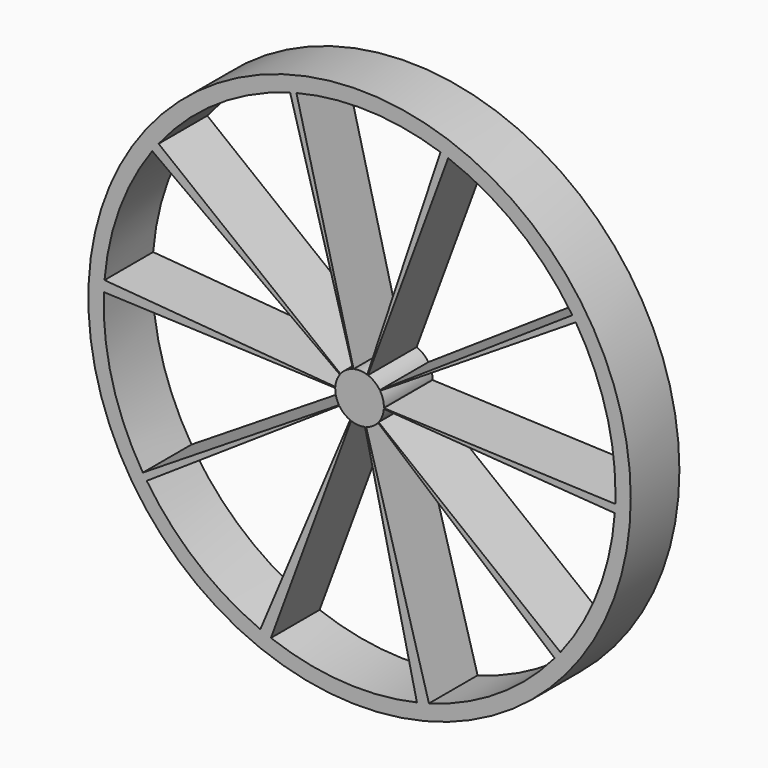
from build123d import *

# Parameters (mm, degrees)
F1_DEPTH = 25.4
F0_R     = 113.2713200319
F2_DEPTH = 25.4


with BuildPart() as f1:
    # F0 (on Front) → F1 (new body)
    with BuildSketch(Plane.XZ):
        with BuildLine():
            Line((0, 0), (8.4491764715, 5.6424300575))
            ThreePointArc((8.4491764715, 5.6424300575), (6.2920375632, 7.9772089921), (3.518990179, 9.53112313))
            Line((3.518990179, 9.53112313), (0, 0))
        make_face()
        with BuildLine():
            Line((-2.5059085691, 9.8461171151), (0, 0))
            Line((0, 0), (3.2131374582, 9.6385345191))
            ThreePointArc((3.2131374582, 9.6385345191), (0.3685319646, 10.1533139512), (-2.5059085691, 9.8461171151))
        make_face()
        with BuildLine():
            Line((-7.9772089921, 6.2920375632), (0, 0))
            Line((0, 0), (-2.7553307558, 9.7792511179))
            ThreePointArc((-2.7553307558, 9.7792511179), (-5.6424300575, 8.4491764715), (-7.9772089921, 6.2920375632))
        make_face()
        with BuildLine():
            Line((-10.1262826145, 0.8270431738), (0, 0))
            Line((0, 0), (-8.2305254154, 5.9568491156))
            ThreePointArc((-8.2305254154, 5.9568491156), (-9.5300486626, 3.5218989889), (-10.1262826145, 0.8270431738))
        make_face()
        with BuildLine():
            Line((-8.6028237663, -5.4052773514), (0, 0))
            Line((0, 0), (-10.1520645288, 0.4014795179))
            ThreePointArc((-10.1520645288, 0.4014795179), (-9.816621877, -2.619071386), (-8.6028237663, -5.4052773514))
        make_face()
        with BuildLine():
            Line((2.2787747925, -9.9011507132), (0, 0))
            Line((0, 0), (-3.518990179, -9.53112313))
            ThreePointArc((-3.518990179, -9.53112313), (-0.6471195054, -10.139370609), (2.2787747925, -9.9011507132))
        make_face()
        with BuildLine():
            Line((7.7452963463, -6.5754075545), (0, 0))
            Line((0, 0), (2.7553307558, -9.7792511179))
            ThreePointArc((2.7553307558, -9.7792511179), (5.4892573067, -8.5494826873), (7.7452963463, -6.5754075545))
        make_face()
        with BuildLine():
            Line((10.1339284401, -0.727388734), (0, 0))
            Line((0, 0), (7.9772089921, -6.2920375632))
            ThreePointArc((7.9772089921, -6.2920375632), (9.4733655012, -3.6716407885), (10.1339284401, -0.727388734))
        make_face()
        with BuildLine():
            Line((-2.7553307558, 9.7792511179), (0, 0))
            Line((0, 0), (-2.5059085691, 9.8461171151))
            ThreePointArc((-2.5059085691, 9.8461171151), (-2.6308321067, 9.8134765719), (-2.7553307558, 9.7792511179))
        make_face()
        with BuildLine():
            Line((-8.2305254154, 5.9568491156), (0, 0))
            Line((0, 0), (-7.9772089921, 6.2920375632))
            ThreePointArc((-7.9772089921, 6.2920375632), (-8.1056000074, 6.1257528942), (-8.2305254154, 5.9568491156))
        make_face()
        with BuildLine():
            Line((-10.1520645288, 0.4014795179), (0, 0))
            Line((0, 0), (-10.1262826145, 0.8270431738))
            ThreePointArc((-10.1262826145, 0.8270431738), (-10.1414060575, 0.6143965965), (-10.1520645288, 0.4014795179))
        make_face()
        with BuildLine():
            Line((-8.4491764715, -5.6424300575), (0, 0))
            Line((0, 0), (-8.6028237663, -5.4052773514))
            ThreePointArc((-8.6028237663, -5.4052773514), (-8.5268246363, -5.5243878956), (-8.4491764715, -5.6424300575))
        make_face()
        with BuildLine():
            Line((-3.9385917856, -9.3655269337), (0, 0))
            Line((0, 0), (-8.4491764715, -5.6424300575))
            ThreePointArc((-8.4491764715, -5.6424300575), (-6.4675778453, -7.8355623164), (-3.9385917856, -9.3655269337))
        make_face()
        with BuildLine():
            Line((2.7553307558, -9.7792511179), (0, 0))
            Line((0, 0), (2.2787747925, -9.9011507132))
            ThreePointArc((2.2787747925, -9.9011507132), (2.517790608, -9.8430854133), (2.7553307558, -9.7792511179))
        make_face()
        with BuildLine():
            Line((-3.518990179, -9.53112313), (0, 0))
            Line((0, 0), (-3.9385917856, -9.3655269337))
            ThreePointArc((-3.9385917856, -9.3655269337), (-3.7297101382, -9.4506540665), (-3.518990179, -9.53112313))
        make_face()
        with BuildLine():
            Line((7.9772089921, -6.2920375632), (0, 0))
            Line((0, 0), (7.7452963463, -6.5754075545))
            ThreePointArc((7.7452963463, -6.5754075545), (7.8625293746, -6.4347674265), (7.9772089921, -6.2920375632))
        make_face()
        with BuildLine():
            ThreePointArc((10.1339284401, -0.727388734), (10.1443053921, -0.5645069636), (10.1520645288, -0.4014795179))
            Line((10.1520645288, -0.4014795179), (0, 0))
            Line((0, 0), (10.1339284401, -0.727388734))
        make_face()
        with BuildLine():
            ThreePointArc((10.1520645288, -0.4014795179), (10.1580159385, -0.2007789674), (10.16, 0))
            ThreePointArc((10.16, 0), (9.7577263861, 2.8306140277), (8.5827606744, 5.4370781864))
            Line((8.5827606744, 5.4370781864), (0, 0))
            Line((0, 0), (10.1520645288, -0.4014795179))
        make_face()
        with BuildLine():
            Line((0, 0), (8.5827606744, 5.4370781864))
            ThreePointArc((8.5827606744, 5.4370781864), (8.5165875257, 5.5401567592), (8.4491764715, 5.6424300575))
            Line((8.4491764715, 5.6424300575), (0, 0))
        make_face()
        with BuildLine():
            Line((3.2131374582, 9.6385345191), (0, 0))
            Line((0, 0), (3.518990179, 9.53112313))
            ThreePointArc((3.518990179, 9.53112313), (3.3664922297, 9.5860487203), (3.2131374582, 9.6385345191))
        make_face()
    extrude(amount=F1_DEPTH)

    # F0 (on Front) → F2 (join)
    with BuildSketch(Plane.XZ):
        Circle(F0_R)
        Polygon((90.5068083934, 60.4411965841), (91.6145348169, 58.0367329004), (104.7544467964, 29.5148519638), (108.7479900799, -4.3006120088), (108.0596985006, -7.7562623179), (102.0965224025, -37.6951021138), (85.4511357641, -67.3997329867), (60.4411965841, -90.5068083934), (29.5148519638, -104.7544467964), (-4.3006120088, -108.7479900799), (-37.6951021138, -102.0965224025), (-67.3997329867, -85.4511357641), (-90.5068083934, -60.4411965841), (-91.7838875883, -57.669130774), (-104.7544467964, -29.5148519638), (-108.7479900799, 4.3006120088), (-107.850128026, 8.8084359851), (-102.0965224025, 37.6951021138), (-87.6655406442, 63.4480026369), (-85.4511357641, 67.3997329867), (-60.4411965841, 90.5068083934), (-29.5148519638, 104.7544467964), (-26.7440517016, 105.0816731443), (4.3006120088, 108.7479900799), (34.2631514946, 102.7800935109), (37.6951021138, 102.0965224025), (67.3997329867, 85.4511357641), align=None, mode=Mode.SUBTRACT)
        with BuildLine():
            ThreePointArc((-8.2305254154, 5.9568491156), (-8.1056000074, 6.1257528942), (-7.9772089921, 6.2920375632))
            Line((-7.9772089921, 6.2920375632), (-83.9123738102, 66.1860318007))
            ThreePointArc((-83.9123738102, 66.1860318007), (-85.2629207095, 64.4368810237), (-86.577012837, 62.6601797971))
            Line((-86.577012837, 62.6601797971), (-8.2305254154, 5.9568491156))
        make_face()
        with BuildLine():
            Line((-28.9833630506, 102.8680803274), (-2.7553307558, 9.7792511179))
            ThreePointArc((-2.7553307558, 9.7792511179), (-2.6308321067, 9.8134765719), (-2.5059085691, 9.8461171151))
            Line((-2.5059085691, 9.8461171151), (-26.3596875538, 103.5714446942))
            ThreePointArc((-26.3596875538, 103.5714446942), (-27.6737600067, 103.2280983602), (-28.9833630506, 102.8680803274))
        make_face()
        with BuildLine():
            ThreePointArc((3.2131374582, 9.6385345191), (3.3664922297, 9.5860487203), (3.518990179, 9.53112313))
            Line((3.518990179, 9.53112313), (37.0163072861, 100.2580185266))
            ThreePointArc((37.0163072861, 100.2580185266), (35.4121792077, 100.8357815844), (33.7990382049, 101.3878804414))
            Line((33.7990382049, 101.3878804414), (3.2131374582, 9.6385345191))
        make_face()
        with BuildLine():
            ThreePointArc((8.4491764715, 5.6424300575), (8.5165875257, 5.5401567592), (8.5827606744, 5.4370781864))
            Line((8.5827606744, 5.4370781864), (90.282180491, 57.1927020673))
            ThreePointArc((90.282180491, 57.1927020673), (89.5861042071, 58.2769870272), (88.8770063774, 59.3528012933))
            Line((88.8770063774, 59.3528012933), (8.4491764715, 5.6424300575))
        make_face()
        with BuildLine():
            Line((106.789709851, -4.2231687065), (10.1520645288, -0.4014795179))
            ThreePointArc((10.1520645288, -0.4014795179), (10.1443053921, -0.5645069636), (10.1339284401, -0.727388734))
            Line((10.1339284401, -0.727388734), (106.5989360787, -7.6514123443))
            ThreePointArc((106.5989360787, -7.6514123443), (106.7080913827, -5.9380567058), (106.789709851, -4.2231687065))
        make_face()
        with BuildLine():
            Line((83.9123738102, -66.1860318007), (7.9772089921, -6.2920375632))
            ThreePointArc((7.9772089921, -6.2920375632), (7.8625293746, -6.4347674265), (7.7452963463, -6.5754075545))
            Line((7.7452963463, -6.5754075545), (81.4728814213, -69.1668047323))
            ThreePointArc((81.4728814213, -69.1668047323), (82.7060572982, -67.687409244), (83.9123738102, -66.1860318007))
        make_face()
        with BuildLine():
            Line((28.9833630506, -102.8680803274), (2.7553307558, -9.7792511179))
            ThreePointArc((2.7553307558, -9.7792511179), (2.517790608, -9.8430854133), (2.2787747925, -9.9011507132))
            Line((2.2787747925, -9.9011507132), (23.9704641575, -104.1503438883))
            ThreePointArc((23.9704641575, -104.1503438883), (26.4846748886, -103.5395541811), (28.9833630506, -102.8680803274))
        make_face()
        with BuildLine():
            Line((-37.0163072861, -100.2580185266), (-3.518990179, -9.53112313))
            ThreePointArc((-3.518990179, -9.53112313), (-3.7297101382, -9.4506540665), (-3.9385917856, -9.3655269337))
            Line((-3.9385917856, -9.3655269337), (-41.4301024994, -98.5161098038))
            ThreePointArc((-41.4301024994, -98.5161098038), (-39.2328735062, -99.4115633134), (-37.0163072861, -100.2580185266))
        make_face()
        with BuildLine():
            Line((-88.8770063774, -59.3528012933), (-8.4491764715, -5.6424300575))
            ThreePointArc((-8.4491764715, -5.6424300575), (-8.5268246363, -5.5243878956), (-8.6028237663, -5.4052773514))
            Line((-8.6028237663, -5.4052773514), (-90.4932244371, -56.8581886358))
            ThreePointArc((-90.4932244371, -56.8581886358), (-89.6937885179, -58.1111141287), (-88.8770063774, -59.3528012933))
        make_face()
        with BuildLine():
            Line((-106.789709851, 4.2231687065), (-10.1520645288, 0.4014795179))
            ThreePointArc((-10.1520645288, 0.4014795179), (-10.1414060575, 0.6143965965), (-10.1262826145, 0.8270431738))
            Line((-10.1262826145, 0.8270431738), (-106.5185095312, 8.6996788006))
            ThreePointArc((-106.5185095312, 8.6996788006), (-106.6775932408, 6.462846457), (-106.789709851, 4.2231687065))
        make_face()
        with BuildLine():
            ThreePointArc((-86.577012837, 62.6601797971), (-85.2629207095, 64.4368810237), (-83.9123738102, 66.1860318007))
            Line((-83.9123738102, 66.1860318007), (-85.4511357641, 67.3997329867))
            Line((-85.4511357641, 67.3997329867), (-87.6655406442, 63.4480026369))
            Line((-87.6655406442, 63.4480026369), (-86.577012837, 62.6601797971))
        make_face()
        with BuildLine():
            Line((-108.7479900799, 4.3006120088), (-106.789709851, 4.2231687065))
            ThreePointArc((-106.789709851, 4.2231687065), (-106.6775932408, 6.462846457), (-106.5185095312, 8.6996788006))
            Line((-106.5185095312, 8.6996788006), (-107.850128026, 8.8084359851))
            Line((-107.850128026, 8.8084359851), (-108.7479900799, 4.3006120088))
        make_face()
        with BuildLine():
            ThreePointArc((-106.5185095312, 8.6996788006), (-100.2467161886, 37.0469050984), (-86.577012837, 62.6601797971))
            Line((-86.577012837, 62.6601797971), (-87.6655406442, 63.4480026369))
            Line((-87.6655406442, 63.4480026369), (-102.0965224025, 37.6951021138))
            Line((-102.0965224025, 37.6951021138), (-107.850128026, 8.8084359851))
            Line((-107.850128026, 8.8084359851), (-106.5185095312, 8.6996788006))
        make_face()
        with BuildLine():
            Line((-91.7838875883, -57.669130774), (-90.4932244371, -56.8581886358))
            ThreePointArc((-90.4932244371, -56.8581886358), (-103.261183869, -27.5500488194), (-106.789709851, 4.2231687065))
            Line((-106.789709851, 4.2231687065), (-108.7479900799, 4.3006120088))
            Line((-108.7479900799, 4.3006120088), (-104.7544467964, -29.5148519638))
            Line((-104.7544467964, -29.5148519638), (-91.7838875883, -57.669130774))
        make_face()
        with BuildLine():
            Line((-90.5068083934, -60.4411965841), (-88.8770063774, -59.3528012933))
            ThreePointArc((-88.8770063774, -59.3528012933), (-89.6937885179, -58.1111141287), (-90.4932244371, -56.8581886358))
            Line((-90.4932244371, -56.8581886358), (-91.7838875883, -57.669130774))
            Line((-91.7838875883, -57.669130774), (-90.5068083934, -60.4411965841))
        make_face()
        with BuildLine():
            Line((-37.6951021138, -102.0965224025), (-37.0163072861, -100.2580185266))
            ThreePointArc((-37.0163072861, -100.2580185266), (-39.2328735062, -99.4115633134), (-41.4301024994, -98.5161098038))
            ThreePointArc((-41.4301024994, -98.5161098038), (-68.0325425023, -82.4223904327), (-88.8770063774, -59.3528012933))
            Line((-88.8770063774, -59.3528012933), (-90.5068083934, -60.4411965841))
            Line((-90.5068083934, -60.4411965841), (-67.3997329867, -85.4511357641))
            Line((-67.3997329867, -85.4511357641), (-37.6951021138, -102.0965224025))
        make_face()
        with BuildLine():
            Line((29.5148519638, -104.7544467964), (28.9833630506, -102.8680803274))
            ThreePointArc((28.9833630506, -102.8680803274), (26.4846748886, -103.5395541811), (23.9704641575, -104.1503438883))
            ThreePointArc((23.9704641575, -104.1503438883), (-6.8070591972, -106.6561823293), (-37.0163072861, -100.2580185266))
            Line((-37.0163072861, -100.2580185266), (-37.6951021138, -102.0965224025))
            Line((-37.6951021138, -102.0965224025), (-4.3006120088, -108.7479900799))
            Line((-4.3006120088, -108.7479900799), (29.5148519638, -104.7544467964))
        make_face()
        with BuildLine():
            Line((85.4511357641, -67.3997329867), (83.9123738102, -66.1860318007))
            ThreePointArc((83.9123738102, -66.1860318007), (82.7060572982, -67.687409244), (81.4728814213, -69.1668047323))
            ThreePointArc((81.4728814213, -69.1668047323), (57.7415749689, -89.9321288755), (28.9833630506, -102.8680803274))
            Line((28.9833630506, -102.8680803274), (29.5148519638, -104.7544467964))
            Line((29.5148519638, -104.7544467964), (60.4411965841, -90.5068083934))
            Line((60.4411965841, -90.5068083934), (85.4511357641, -67.3997329867))
        make_face()
        with BuildLine():
            Line((108.0596985006, -7.7562623179), (106.5989360787, -7.6514123443))
            ThreePointArc((106.5989360787, -7.6514123443), (99.6504652153, -38.6220411987), (83.9123738102, -66.1860318007))
            Line((83.9123738102, -66.1860318007), (85.4511357641, -67.3997329867))
            Line((85.4511357641, -67.3997329867), (102.0965224025, -37.6951021138))
            Line((102.0965224025, -37.6951021138), (108.0596985006, -7.7562623179))
        make_face()
        with BuildLine():
            Line((91.6145348169, 58.0367329004), (90.282180491, 57.1927020673))
            ThreePointArc((90.282180491, 57.1927020673), (102.6416613707, 29.7752688491), (106.8731831844, 0))
            ThreePointArc((106.8731831844, 0), (106.8523128133, -2.1119967875), (106.789709851, -4.2231687065))
            Line((106.789709851, -4.2231687065), (108.7479900799, -4.3006120088))
            Line((108.7479900799, -4.3006120088), (104.7544467964, 29.5148519638))
            Line((104.7544467964, 29.5148519638), (91.6145348169, 58.0367329004))
        make_face()
        with BuildLine():
            Line((108.7479900799, -4.3006120088), (106.789709851, -4.2231687065))
            ThreePointArc((106.789709851, -4.2231687065), (106.7080913827, -5.9380567058), (106.5989360787, -7.6514123443))
            Line((106.5989360787, -7.6514123443), (108.0596985006, -7.7562623179))
            Line((108.0596985006, -7.7562623179), (108.7479900799, -4.3006120088))
        make_face()
        with BuildLine():
            ThreePointArc((88.8770063774, 59.3528012933), (89.5861042071, 58.2769870272), (90.282180491, 57.1927020673))
            Line((90.282180491, 57.1927020673), (91.6145348169, 58.0367329004))
            Line((91.6145348169, 58.0367329004), (90.5068083934, 60.4411965841))
            Line((90.5068083934, 60.4411965841), (88.8770063774, 59.3528012933))
        make_face()
        with BuildLine():
            ThreePointArc((37.0163072861, 100.2580185266), (66.1860318007, 83.9123738102), (88.8770063774, 59.3528012933))
            Line((88.8770063774, 59.3528012933), (90.5068083934, 60.4411965841))
            Line((90.5068083934, 60.4411965841), (67.3997329867, 85.4511357641))
            Line((67.3997329867, 85.4511357641), (37.6951021138, 102.0965224025))
            Line((37.6951021138, 102.0965224025), (37.0163072861, 100.2580185266))
        make_face()
        with BuildLine():
            ThreePointArc((33.7990382049, 101.3878804414), (35.4121792077, 100.8357815844), (37.0163072861, 100.2580185266))
            Line((37.0163072861, 100.2580185266), (37.6951021138, 102.0965224025))
            Line((37.6951021138, 102.0965224025), (34.2631514946, 102.7800935109))
            Line((34.2631514946, 102.7800935109), (33.7990382049, 101.3878804414))
        make_face()
        with BuildLine():
            Line((-26.7440517016, 105.0816731443), (-26.3596875538, 103.5714446942))
            ThreePointArc((-26.3596875538, 103.5714446942), (3.8765929293, 106.8028525426), (33.7990382049, 101.3878804414))
            Line((33.7990382049, 101.3878804414), (34.2631514946, 102.7800935109))
            Line((34.2631514946, 102.7800935109), (4.3006120088, 108.7479900799))
            Line((4.3006120088, 108.7479900799), (-26.7440517016, 105.0816731443))
        make_face()
        with BuildLine():
            ThreePointArc((-83.9123738102, 66.1860318007), (-59.3528012933, 88.8770063774), (-28.9833630506, 102.8680803274))
            Line((-28.9833630506, 102.8680803274), (-29.5148519638, 104.7544467964))
            Line((-29.5148519638, 104.7544467964), (-60.4411965841, 90.5068083934))
            Line((-60.4411965841, 90.5068083934), (-85.4511357641, 67.3997329867))
            Line((-85.4511357641, 67.3997329867), (-83.9123738102, 66.1860318007))
        make_face()
        with BuildLine():
            Line((-29.5148519638, 104.7544467964), (-28.9833630506, 102.8680803274))
            ThreePointArc((-28.9833630506, 102.8680803274), (-27.6737600067, 103.2280983602), (-26.3596875538, 103.5714446942))
            Line((-26.3596875538, 103.5714446942), (-26.7440517016, 105.0816731443))
            Line((-26.7440517016, 105.0816731443), (-29.5148519638, 104.7544467964))
        make_face()
    extrude(amount=F2_DEPTH)


solid = f1.part
